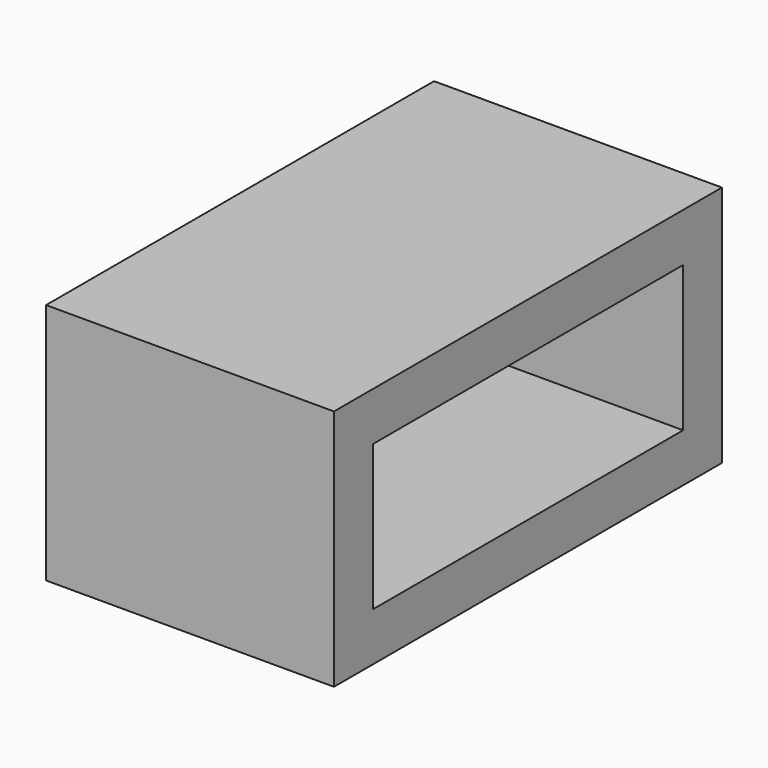
from build123d import *

# Parameters (mm, degrees)
F0_W     = 16
F0_H     = 8
F1_DEPTH = 9.5
F2_R     = 1.25
F3_DEPTH = 1.9
F4_W     = 12.8
F4_H     = 4.8
F6_DEPTH = 8.5


# Not quite as in the source:
# - a feature names something its author has since deleted; it is built from what else it names


with BuildPart() as f1:
    # F0 (on Right) → F1 (new body)
    with BuildSketch(Plane.YZ):
        with Locations((41.7828243226, 21.9434328547)):
            Rectangle(F0_W, F0_H)
    extrude(amount=F1_DEPTH)

    # F2 (on face) → F3 (join)
    with BuildSketch(Plane(origin=(0, 0, 0), x_dir=(0, -1, 0), z_dir=(-1, 0, 0))):
        with Locations((-44.8828243226, 21.9434328547)):
            Circle(F2_R)
        with Locations((-38.6828243226, 21.9434328547)):
            Circle(F2_R)
    extrude(amount=F3_DEPTH)

    # F4 (on face) → F6 (cut)
    with BuildSketch(Plane.YZ.offset(9.5)):
        with Locations((41.7828243226, 21.9434328547)):
            Rectangle(F4_W, F4_H)
    extrude(amount=-F6_DEPTH, mode=Mode.SUBTRACT)


solid = f1.part
